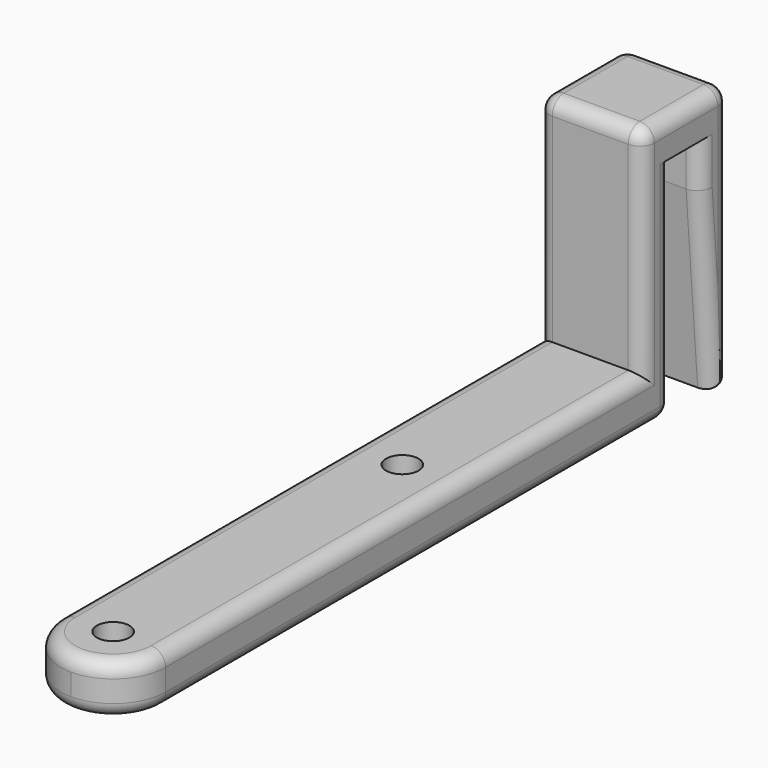
from build123d import *

# Parameters (mm, degrees)
F2_R          = 2.25
F7_DEPTH      = 7
F10_R         = 4
F10_R_2       = 2.25
F11_DEPTH     = 2.5
F12_SIZE2     = 1.74999
F12_SIZE      = 2.09999
F12_2_SIZE2   = 1.74999
F12_2_SIZE    = 2.09999
F14_W         = 14.5
F14_H         = 25.25
F15_DEPTH     = 7
F16_W         = 14.5
F16_H         = 29.5
F16_H_2       = 7
F17_DEPTH     = 5
F18_W         = 14.5
F18_H         = 5
F19_DEPTH     = 10
F20_W         = 14.5
F20_H         = 5
F21_DEPTH     = 31.5
F22_SIZE2     = 2
F22_SIZE      = 25
F23_T1_DEPTH  = 11
F23_T3_DEPTH  = 27.5
F23_T5_DEPTH  = 29.5
F23_T7_DEPTH  = 11.5
F23_T9_DEPTH  = 39.5
F23_T11_DEPTH = 35.079872408
F23_T13_DEPTH = 82.5
F23_T15_DEPTH = 85.5
F23_T17_DEPTH = 5
F23_T19_DEPTH = 10.5
F23_T21_DEPTH = 17.5
F23_T23_DEPTH = 92.4999999229
F23_T25_DEPTH = 82.4999999229
F23_S29_W     = 2
F23_S29_H     = 2
F23_T30_DEPTH = 2
F23_S35_W     = 2
F23_S35_H     = 2
F23_T36_DEPTH = 2
F23_S41_W     = 2
F23_S41_H     = 2
F23_T42_DEPTH = 2
F23_S47_W     = 2
F23_S47_H     = 2
F23_T48_DEPTH = 2
F23_S53_W     = 2
F23_S53_H     = 2
F23_T54_DEPTH = 2
F23_T58_ANGLE = 180.0000006096
F23_T60_ANGLE = 180.0000006096
F23_T65_DEPTH = 32.5
F23_T69_DEPTH = 87.5
F23_T76_DEPTH = 32.5
F23_T80_DEPTH = 87.4999999229
F23_T87_DEPTH = 16.5
F23_T91_DEPTH = 10
F24_R         = 0.99999


# Not quite as in the source:
# - a fillet or chamfer that OpenCascade refuses, or shapes differently, is made with other operations: its cross-section is extruded or revolved along the edge and cut away or added
# - a fillet or chamfer is up to 0.001 mm smaller than in the source, because OpenCascade refuses the exact size


with BuildPart() as f7:
    # F2 (on Top) → F7 (new body)
    with BuildSketch(Plane.XY):
        with BuildLine():
            Line((-3.2788694371, 52.1037624441), (-17.7788694371, 52.1037624441))
            Line((-17.7788694371, 52.1037624441), (-17.7788694371, -5.1462374788))
            ThreePointArc((-17.7788694371, -5.1462374788), (-10.5288693985, 2.1037624441), (-3.2788694371, -5.1462375559))
            Line((-3.2788694371, -5.1462375559), (-3.2788694371, 52.1037624441))
        make_face()
        with Locations((-10.5288694371, 44.8537624441)):
            Circle(F2_R, mode=Mode.SUBTRACT)
        with BuildLine():
            ThreePointArc((-3.2788694371, -5.1462375559), (-10.5288693985, 2.1037624441), (-17.7788694371, -5.1462374788))
            ThreePointArc((-17.7788694371, -5.1462374788), (-15.6553936279, -10.2727616922), (-10.5288694371, -12.3962375559))
            ThreePointArc((-10.5288694371, -12.3962375559), (-5.4023452735, -10.2727617195), (-3.2788694371, -5.1462375559))
        make_face()
        with Locations((-10.5288694371, -5.1462375559)):
            Circle(F2_R, mode=Mode.SUBTRACT)
    extrude(amount=F7_DEPTH)

    # F10 (on face) → F11 (cut)
    with BuildSketch(Plane(origin=(0, 0, 0), x_dir=(1, 0, 0), z_dir=(0, 0, -1))):
        with Locations((-10.5288694371, 5.1462375559)):
            Circle(F10_R)
        with Locations((-10.5288694371, 5.1462375559)):
            Circle(F10_R_2, mode=Mode.SUBTRACT)
        with Locations((-10.5288694371, -44.8537624441)):
            Circle(F10_R)
        with Locations((-10.5288694371, -44.8537624441)):
            Circle(F10_R_2, mode=Mode.SUBTRACT)
    extrude(amount=-F11_DEPTH, mode=Mode.SUBTRACT)

    # F12 (size 2.1 and 1.75 in the source; OpenCascade refuses exactly that, so slightly less here)
    f12_edges = [f7.edges().sort_by_distance(p)[0] for p in [
        (-14.528869, -5.146238, 2.5),
    ]]
    f12_side = f7.faces().sort_by_distance((-14.528869, -5.146238, 1.25))[0]
    chamfer(f12_edges, length=F12_SIZE, length2=F12_SIZE2, reference=f12_side)

    # F12#2 (size 2.1 and 1.75 in the source; OpenCascade refuses exactly that, so slightly less here)
    f12_2_edges = [f7.edges().sort_by_distance(p)[0] for p in [
        (-14.528869, 44.853762, 2.5),
    ]]
    f12_2_side = f7.faces().sort_by_distance((-14.528869, 44.853762, 1.25))[0]
    chamfer(f12_2_edges, length=F12_2_SIZE, length2=F12_2_SIZE2, reference=f12_2_side)

    # F14 (on face) → F15 (join)
    with BuildSketch(Plane.XY.offset(7)):
        with Locations((-10.5288694371, 64.7287624441)):
            Rectangle(F14_W, F14_H)
    extrude(amount=-F15_DEPTH)

    # F16 (on face) → F17 (join)
    with BuildSketch(Plane(origin=(0, 77.3537624441, 0), x_dir=(-1, 0, 0), z_dir=(0, 1, 0))):
        with Locations((10.5288694371, 21.75)):
            Rectangle(F16_W, F16_H)
        with Locations((10.5288694371, 3.5)):
            Rectangle(F16_W, F16_H_2)
    extrude(amount=F17_DEPTH)

    # F18 (on face) → F19 (join)
    with BuildSketch(Plane(origin=(0, 82.3537624441, 0), x_dir=(-1, 0, 0), z_dir=(0, 1, 0))):
        with Locations((10.5288694371, 34)):
            Rectangle(F18_W, F18_H)
    extrude(amount=F19_DEPTH)

    # F20 (on face) → F21 (join)
    with BuildSketch(Plane(origin=(0, 0, 31.5), x_dir=(1, 0, 0), z_dir=(0, 0, -1))):
        with Locations((-10.5288694371, -89.8537624441)):
            Rectangle(F20_W, F20_H)
    extrude(amount=F21_DEPTH)

    # F22
    f22_edges = [f7.edges().sort_by_distance(p)[0] for p in [
        (-10.528869, 87.353762, 0),
    ]]
    f22_side = f7.faces().sort_by_distance((-10.528869, 87.353762, 15.75))[0]
    chamfer(f22_edges, length=F22_SIZE, length2=F22_SIZE2, reference=f22_side)

    # F23: fillet of radius 2 on 17 edges, made by hand

    # F23_s2 → F23_t1 (cut)
    with BuildSketch(Plane.XZ.offset(-90.3537624441)):
        with BuildLine():
            ThreePointArc((-3.2788694371, 34.5), (-3.8646558747, 35.9142135624), (-5.2788694371, 36.5))
            Line((-5.2788694371, 36.5), (-3.2788694371, 36.5))
            Line((-3.2788694371, 36.5), (-3.2788694371, 34.5))
        make_face()
        with BuildLine():
            ThreePointArc((-17.7788694371, 34.5), (-17.1930829994, 35.9142135624), (-15.7788694371, 36.5))
            Line((-15.7788694371, 36.5), (-17.7788694371, 36.5))
            Line((-17.7788694371, 36.5), (-17.7788694371, 34.5))
        make_face()
    extrude(amount=F23_T1_DEPTH, mode=Mode.SUBTRACT)

    # F23_s4 → F23_t3 (cut)
    with BuildSketch(Plane.XY.offset(7)):
        with BuildLine():
            ThreePointArc((-3.2788694371, 79.3537624441), (-3.8646558747, 77.9395488817), (-5.2788694371, 77.3537624441))
            Line((-5.2788694371, 77.3537624441), (-3.2788694371, 77.3537624441))
            Line((-3.2788694371, 77.3537624441), (-3.2788694371, 79.3537624441))
        make_face()
        with BuildLine():
            ThreePointArc((-17.7788694371, 79.3537624441), (-17.1930829994, 77.9395488817), (-15.7788694371, 77.3537624441))
            Line((-15.7788694371, 77.3537624441), (-17.7788694371, 77.3537624441))
            Line((-17.7788694371, 77.3537624441), (-17.7788694371, 79.3537624441))
        make_face()
    extrude(amount=F23_T3_DEPTH, mode=Mode.SUBTRACT)

    # F23_s6 → F23_t5 (cut)
    with BuildSketch(Plane.XY.offset(2)):
        with BuildLine():
            ThreePointArc((-3.2788694371, 80.3537624441), (-3.8646558747, 81.7679760065), (-5.2788694371, 82.3537624441))
            Line((-5.2788694371, 82.3537624441), (-3.2788694371, 82.3537624441))
            Line((-3.2788694371, 82.3537624441), (-3.2788694371, 80.3537624441))
        make_face()
    extrude(amount=F23_T5_DEPTH, mode=Mode.SUBTRACT)

    # F23_s8 → F23_t7 (cut)
    with BuildSketch(Plane.XY.offset(20)):
        with BuildLine():
            ThreePointArc((-3.2788694371, 89.3537624441), (-3.8646558747, 87.9395488817), (-5.2788694371, 87.3537624441))
            Line((-5.2788694371, 87.3537624441), (-3.2788694371, 87.3537624441))
            Line((-3.2788694371, 87.3537624441), (-3.2788694371, 89.3537624441))
        make_face()
        with BuildLine():
            ThreePointArc((-17.7788694371, 89.3537624441), (-17.1930829994, 87.9395488817), (-15.7788694371, 87.3537624441))
            Line((-15.7788694371, 87.3537624441), (-17.7788694371, 87.3537624441))
            Line((-17.7788694371, 87.3537624441), (-17.7788694371, 89.3537624441))
        make_face()
    extrude(amount=F23_T7_DEPTH, mode=Mode.SUBTRACT)

    # F23_s10 → F23_t9 (cut)
    with BuildSketch(Plane.XY.offset(-5)):
        with BuildLine():
            ThreePointArc((-5.2788694371, 92.3537624441), (-3.8646558747, 91.7679760065), (-3.2788694371, 90.3537624441))
            Line((-3.2788694371, 90.3537624441), (-3.2788694371, 92.3537624441))
            Line((-3.2788694371, 92.3537624441), (-5.2788694371, 92.3537624441))
        make_face()
        with BuildLine():
            ThreePointArc((-17.7788694371, 90.3537624441), (-17.1930829994, 91.7679760065), (-15.7788694371, 92.3537624441))
            Line((-15.7788694371, 92.3537624441), (-17.7788694371, 92.3537624441))
            Line((-17.7788694371, 92.3537624441), (-17.7788694371, 90.3537624441))
        make_face()
    extrude(amount=F23_T9_DEPTH, mode=Mode.SUBTRACT)

    # F23_s12 → F23_t11 (cut)
    with BuildSketch(Plane(origin=(0, -1.8304986873, 22.8812335911), x_dir=(1, 0, 0), z_dir=(0, 0.0797452223, -0.9968152785))):
        with BuildLine():
            ThreePointArc((-5.2788694371, -89.069195599), (-3.8646558747, -89.6549820366), (-3.2788694371, -91.069195599))
            Line((-3.2788694371, -91.069195599), (-3.2788694371, -89.069195599))
            Line((-3.2788694371, -89.069195599), (-5.2788694371, -89.069195599))
        make_face()
        with BuildLine():
            ThreePointArc((-17.7788694371, -91.069195599), (-17.1930829994, -89.6549820366), (-15.7788694371, -89.069195599))
            Line((-15.7788694371, -89.069195599), (-17.7788694371, -89.069195599))
            Line((-17.7788694371, -89.069195599), (-17.7788694371, -91.069195599))
        make_face()
    extrude(amount=F23_T11_DEPTH, mode=Mode.SUBTRACT)

    # F23_s14 → F23_t13 (cut)
    with BuildSketch(Plane.XZ.offset(-77.3537624441)):
        with BuildLine():
            ThreePointArc((-3.2788694371, 5), (-3.8646558747, 6.4142135624), (-5.2788694371, 7))
            Line((-5.2788694371, 7), (-3.2788694371, 7))
            Line((-3.2788694371, 7), (-3.2788694371, 5))
        make_face()
    extrude(amount=F23_T13_DEPTH, mode=Mode.SUBTRACT)

    # F23_s16 → F23_t15 (cut)
    with BuildSketch(Plane.XZ.offset(-80.3537624441)):
        with BuildLine():
            ThreePointArc((-3.2788694371, 2), (-3.8646558747, 0.5857864376), (-5.2788694371, 0))
            Line((-5.2788694371, 0), (-3.2788694371, 0))
            Line((-3.2788694371, 0), (-3.2788694371, 2))
        make_face()
    extrude(amount=F23_T15_DEPTH, mode=Mode.SUBTRACT)

    # F23_s18 → F23_t17 (cut)
    with BuildSketch(Plane.XZ.offset(-87.3537624441)):
        with BuildLine():
            ThreePointArc((-17.7788694371, 33.5), (-17.1930829994, 32.0857864376), (-15.7788694371, 31.5))
            Line((-15.7788694371, 31.5), (-17.7788694371, 31.5))
            Line((-17.7788694371, 31.5), (-17.7788694371, 33.5))
        make_face()
    extrude(amount=F23_T17_DEPTH, mode=Mode.SUBTRACT)

    # F23_s20 → F23_t19 (cut)
    with BuildSketch(Plane.YZ.offset(-15.7788694371)):
        with BuildLine():
            ThreePointArc((79.3537624441, 36.5), (77.9395488817, 35.9142135624), (77.3537624441, 34.5))
            Line((77.3537624441, 34.5), (77.3537624441, 36.5))
            Line((77.3537624441, 36.5), (79.3537624441, 36.5))
        make_face()
        with BuildLine():
            ThreePointArc((92.3537624441, 34.5), (91.7679760065, 35.9142135624), (90.3537624441, 36.5))
            Line((90.3537624441, 36.5), (92.3537624441, 36.5))
            Line((92.3537624441, 36.5), (92.3537624441, 34.5))
        make_face()
    extrude(amount=F23_T19_DEPTH, mode=Mode.SUBTRACT)

    # F23_s22 → F23_t21 (cut)
    with BuildSketch(Plane.YZ.offset(-22.7788694371)):
        with BuildLine():
            ThreePointArc((82.3537624441, 2), (81.7679760065, 0.5857864376), (80.3537624441, 0))
            Line((80.3537624441, 0), (82.3537624441, 0))
            Line((82.3537624441, 0), (82.3537624441, 2))
        make_face()
    extrude(amount=F23_T21_DEPTH, mode=Mode.SUBTRACT)

    # F23_s24 → F23_t23 (cut)
    with BuildSketch(Plane.XZ.offset(-87.3537624441)):
        with BuildLine():
            ThreePointArc((-17.7788694371, 2), (-17.1930829994, 0.5857864376), (-15.7788694371, 0))
            Line((-15.7788694371, 0), (-17.7788694371, 0))
            Line((-17.7788694371, 0), (-17.7788694371, 2))
        make_face()
    extrude(amount=F23_T23_DEPTH, mode=Mode.SUBTRACT)

    # F23_s26 → F23_t25 (cut)
    with BuildSketch(Plane.XZ.offset(-77.3537624441)):
        with BuildLine():
            ThreePointArc((-17.7788694371, 5), (-17.1930829994, 6.4142135624), (-15.7788694371, 7))
            Line((-15.7788694371, 7), (-17.7788694371, 7))
            Line((-17.7788694371, 7), (-17.7788694371, 5))
        make_face()
    extrude(amount=F23_T25_DEPTH, mode=Mode.SUBTRACT)


with BuildPart() as f23_tool28:
    # F23_s29 → F23_t30 (new body)
    with BuildSketch(Plane.XY.offset(34.5)):
        with Locations((-4.2788694371, 91.3537624441)):
            Rectangle(F23_S29_W, F23_S29_H)
    extrude(amount=F23_T30_DEPTH)

    # F23_s31 → F23_t32 (revolve, cut)
    with BuildSketch(Plane(origin=(-5.2788694371, 90.3537624441, 34.5), x_dir=(-0.7071067812, -0.7071067812, 0), z_dir=(-0.7071067812, 0.7071067812, 0))):
        with BuildLine():
            ThreePointArc((0, -2), (2, 0), (0, 2))
            Line((0, 2), (0, -2))
        make_face()
    revolve(axis=Axis((-5.2788694371, 90.3537624441, 34.5), (0, 0, 1)), mode=Mode.SUBTRACT)


with BuildPart() as f7_1:
    add(f7.part)

    # F23_t27: cut F23_tool28
    add(f23_tool28.part, mode=Mode.SUBTRACT)


with BuildPart() as f23_tool34:
    # F23_s35 → F23_t36 (new body)
    with BuildSketch(Plane.XY.offset(34.5)):
        with Locations((-4.2788694371, 78.3537624441)):
            Rectangle(F23_S35_W, F23_S35_H)
    extrude(amount=F23_T36_DEPTH)

    # F23_s37 → F23_t38 (revolve, cut)
    with BuildSketch(Plane(origin=(-5.2788694371, 79.3537624441, 34.5), x_dir=(-0.7071067812, 0.7071067812, 0), z_dir=(0.7071067812, 0.7071067812, 0))):
        with BuildLine():
            ThreePointArc((0, -2), (2, 0), (0, 2))
            Line((0, 2), (0, -2))
        make_face()
    revolve(axis=Axis((-5.2788694371, 79.3537624441, 34.5), (0, 0, 1)), mode=Mode.SUBTRACT)


with BuildPart() as f7_2:
    add(f7_1.part)

    # F23_t33: cut F23_tool34
    add(f23_tool34.part, mode=Mode.SUBTRACT)


with BuildPart() as f23_tool40:
    # F23_s41 → F23_t42 (new body)
    with BuildSketch(Plane.XY.offset(2)):
        with Locations((-4.2788694371, 81.3537624441)):
            Rectangle(F23_S41_W, F23_S41_H)
    extrude(amount=-F23_T42_DEPTH)

    # F23_s43 → F23_t44 (revolve, cut)
    with BuildSketch(Plane(origin=(-5.2788694371, 80.3537624441, 2), x_dir=(-0.7071067812, -0.7071067812, 0), z_dir=(0.7071067812, -0.7071067812, 0))):
        with BuildLine():
            ThreePointArc((0, -2), (2, 0), (0, 2))
            Line((0, 2), (0, -2))
        make_face()
    revolve(axis=Axis((-5.2788694371, 80.3537624441, 2), (0, 0, -1)), mode=Mode.SUBTRACT)


with BuildPart() as f7_3:
    add(f7_2.part)

    # F23_t39: cut F23_tool40
    add(f23_tool40.part, mode=Mode.SUBTRACT)


with BuildPart() as f23_tool46:
    # F23_s47 → F23_t48 (new body)
    with BuildSketch(Plane.YZ.offset(-15.7788694371)):
        with Locations((78.3537624441, 35.5)):
            Rectangle(F23_S47_W, F23_S47_H)
    extrude(amount=-F23_T48_DEPTH)

    # F23_s49 → F23_t50 (revolve, cut)
    with BuildSketch(Plane(origin=(-15.7788694371, 79.3537624441, 34.5), x_dir=(0, 0.7071067812, -0.7071067812), z_dir=(0, 0.7071067812, 0.7071067812))):
        with BuildLine():
            ThreePointArc((0, -2), (2, 0), (0, 2))
            Line((0, 2), (0, -2))
        make_face()
    revolve(axis=Axis((-15.7788694371, 79.3537624441, 34.5), (-1, 0, 0)), mode=Mode.SUBTRACT)


with BuildPart() as f7_4:
    add(f7_3.part)

    # F23_t45: cut F23_tool46
    add(f23_tool46.part, mode=Mode.SUBTRACT)


with BuildPart() as f23_tool52:
    # F23_s53 → F23_t54 (new body)
    with BuildSketch(Plane.YZ.offset(-15.7788694371)):
        with Locations((91.3537624441, 35.5)):
            Rectangle(F23_S53_W, F23_S53_H)
    extrude(amount=-F23_T54_DEPTH)

    # F23_s55 → F23_t56 (revolve, cut)
    with BuildSketch(Plane(origin=(-15.7788694371, 90.3537624441, 34.5), x_dir=(0, -0.7071067812, -0.7071067812), z_dir=(0, 0.7071067812, -0.7071067812))):
        with BuildLine():
            ThreePointArc((0, -2), (2, 0), (0, 2))
            Line((0, 2), (0, -2))
        make_face()
    revolve(axis=Axis((-15.7788694371, 90.3537624441, 34.5), (-1, 0, 0)), mode=Mode.SUBTRACT)


with BuildPart() as f7_5:
    add(f7_4.part)

    # F23_t51: cut F23_tool52
    add(f23_tool52.part, mode=Mode.SUBTRACT)

    # F23_s57 → F23_t58 (revolve, cut)
    with BuildSketch(Plane.XZ.offset(5.1462375559)):
        with BuildLine():
            ThreePointArc((-15.7788694371, 0), (-17.1930829994, 0.5857864376), (-17.7788694371, 2))
            Line((-17.7788694371, 2), (-17.7788694371, 0))
            Line((-17.7788694371, 0), (-15.7788694371, 0))
        make_face()
    revolve(axis=Axis((-10.5288694371, -5.1462375559, 0), (0, 0, 1)), revolution_arc=F23_T58_ANGLE, mode=Mode.SUBTRACT)

    # F23_s59 → F23_t60 (revolve, cut)
    with BuildSketch(Plane.XZ.offset(5.1462375559)):
        with BuildLine():
            ThreePointArc((-17.7788694371, 5), (-17.1930829994, 6.4142135624), (-15.7788694371, 7))
            Line((-15.7788694371, 7), (-17.7788694371, 7))
            Line((-17.7788694371, 7), (-17.7788694371, 5))
        make_face()
    revolve(axis=Axis((-10.5288694371, -5.1462375559, 7), (0, 0, 1)), revolution_arc=F23_T60_ANGLE, mode=Mode.SUBTRACT)


with BuildPart() as f23_tool63:
    # F23_s64 → F23_t65 (new body)
    with BuildSketch(Plane.XY.offset(34.5)):
        with BuildLine():
            ThreePointArc((-3.2788694371, 79.3537624441), (-3.8646558747, 77.9395488817), (-5.2788694371, 77.3537624441))
            Line((-5.2788694371, 77.3537624441), (-3.2788694371, 77.3537624441))
            Line((-3.2788694371, 77.3537624441), (-3.2788694371, 79.3537624441))
        make_face()
    extrude(amount=-F23_T65_DEPTH)

    split(bisect_by=Plane.XY.offset(7), keep=Keep.BOTTOM)


with BuildPart() as f23_tool67:
    # F23_s68 → F23_t69 (new body)
    with BuildSketch(Plane.XZ.offset(-82.3537624441)):
        with BuildLine():
            ThreePointArc((-3.2788694371, 5), (-3.8646558747, 6.4142135624), (-5.2788694371, 7))
            Line((-5.2788694371, 7), (-3.2788694371, 7))
            Line((-3.2788694371, 7), (-3.2788694371, 5))
        make_face()
    extrude(amount=F23_T69_DEPTH)

    split(bisect_by=Plane.XZ.offset(-77.3537624441), keep=Keep.BOTTOM)


with BuildPart() as f23_tool63_1:
    add(f23_tool63.part)

    # F23_t71: intersect F23_tool67
    add(f23_tool67.part, mode=Mode.INTERSECT)


with BuildPart() as f7_6:
    add(f7_5.part)

    # F23_t61: cut F23_tool63
    add(f23_tool63_1.part, mode=Mode.SUBTRACT)


with BuildPart() as f23_tool74:
    # F23_s75 → F23_t76 (new body)
    with BuildSketch(Plane.XY.offset(2)):
        with BuildLine():
            ThreePointArc((-17.7788694371, 79.3537624441), (-17.1930829994, 77.9395488817), (-15.7788694371, 77.3537624441))
            Line((-15.7788694371, 77.3537624441), (-17.7788694371, 77.3537624441))
            Line((-17.7788694371, 77.3537624441), (-17.7788694371, 79.3537624441))
        make_face()
    extrude(amount=F23_T76_DEPTH)

    split(bisect_by=Plane.XY.offset(7), keep=Keep.BOTTOM)


with BuildPart() as f23_tool78:
    # F23_s79 → F23_t80 (new body)
    with BuildSketch(Plane.XZ.offset(5.1462374788)):
        with BuildLine():
            ThreePointArc((-17.7788694371, 5), (-17.1930829994, 6.4142135624), (-15.7788694371, 7))
            Line((-15.7788694371, 7), (-17.7788694371, 7))
            Line((-17.7788694371, 7), (-17.7788694371, 5))
        make_face()
    extrude(amount=-F23_T80_DEPTH)

    split(bisect_by=Plane.XZ.offset(-77.3537624441), keep=Keep.BOTTOM)


with BuildPart() as f23_tool74_1:
    add(f23_tool74.part)

    # F23_t82: intersect F23_tool78
    add(f23_tool78.part, mode=Mode.INTERSECT)


with BuildPart() as f7_7:
    add(f7_6.part)

    # F23_t72: cut F23_tool74
    add(f23_tool74_1.part, mode=Mode.SUBTRACT)


with BuildPart() as f23_tool85:
    # F23_s86 → F23_t87 (new body)
    with BuildSketch(Plane.XY.offset(36.5)):
        with BuildLine():
            ThreePointArc((-17.7788694371, 89.3537624441), (-17.1930829994, 87.9395488817), (-15.7788694371, 87.3537624441))
            Line((-15.7788694371, 87.3537624441), (-17.7788694371, 87.3537624441))
            Line((-17.7788694371, 87.3537624441), (-17.7788694371, 89.3537624441))
        make_face()
    extrude(amount=-F23_T87_DEPTH)

    split(bisect_by=Plane.XY.offset(31.5), keep=Keep.TOP)


with BuildPart() as f23_tool89:
    # F23_s90 → F23_t91 (new body)
    with BuildSketch(Plane.XZ.offset(-82.3537624441)):
        with BuildLine():
            ThreePointArc((-17.7788694371, 33.5), (-17.1930829994, 32.0857864376), (-15.7788694371, 31.5))
            Line((-15.7788694371, 31.5), (-17.7788694371, 31.5))
            Line((-17.7788694371, 31.5), (-17.7788694371, 33.5))
        make_face()
    extrude(amount=-F23_T91_DEPTH)

    split(bisect_by=Plane.XZ.offset(-87.3537624441), keep=Keep.BOTTOM)


with BuildPart() as f23_tool85_1:
    add(f23_tool85.part)

    # F23_t93: intersect F23_tool89
    add(f23_tool89.part, mode=Mode.INTERSECT)


with BuildPart() as f7_8:
    add(f7_7.part)

    # F23_t83: cut F23_tool85
    add(f23_tool85_1.part, mode=Mode.SUBTRACT)

    # F24 (radius 1 in the source; OpenCascade refuses exactly that, so slightly less here)
    f24_edges = [f7_8.edges().sort_by_distance(p)[0] for p in [
        (-10.528869, 92.353762, 0),
    ]]
    fillet(f24_edges, radius=F24_R)


solid = f7_8.part
